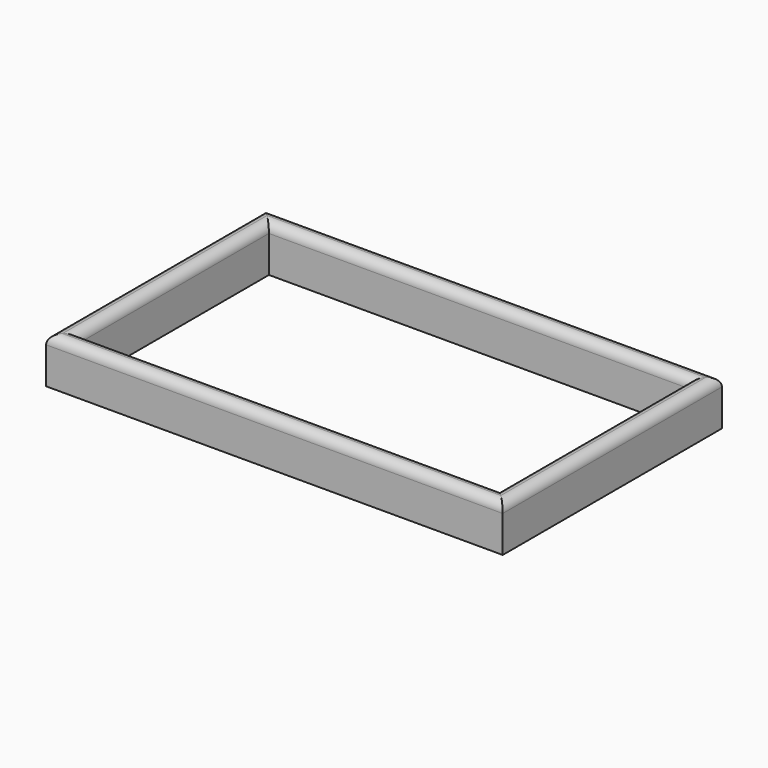
from build123d import *

# Parameters (mm, degrees)
F0_W     = 250
F0_H     = 150
F0_W_2   = 230
F0_H_2   = 130
F1_DEPTH = 25
F2_R     = 4.99999


# Not quite as in the source:
# - a fillet or chamfer is up to 0.001 mm smaller than in the source, because OpenCascade refuses the exact size


with BuildPart() as f1:
    # F0 (on Top) → F1 (new body)
    with BuildSketch(Plane.XY):
        Rectangle(F0_W, F0_H)
        Rectangle(F0_W_2, F0_H_2, mode=Mode.SUBTRACT)
    extrude(amount=F1_DEPTH)

    # F2 (radius 5 in the source; OpenCascade refuses exactly that, so slightly less here)
    f2_edges = [f1.edges().sort_by_distance(p)[0] for p in [
        (0, 75, 25),
        (-125, 0, 25),
        (0, -75, 25),
        (125, 0, 25),
        (-115, 0, 25),
        (0, 65, 25),
        (115, 0, 25),
        (0, -65, 25),
    ]]
    fillet(f2_edges, radius=F2_R)


solid = f1.part
